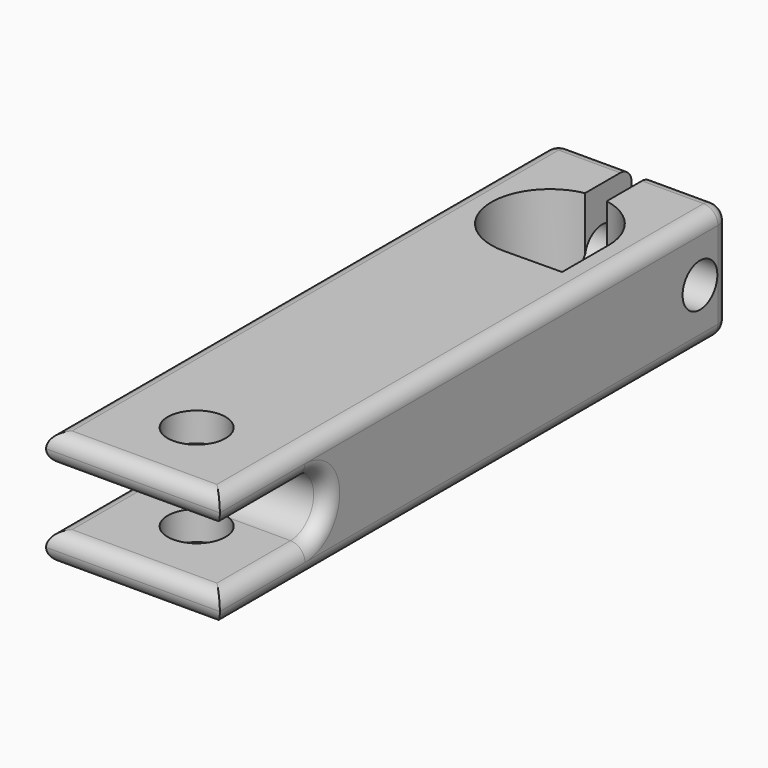
from build123d import *

# Parameters (mm, degrees)
F0_W      = 38.1
F0_H      = 139.7
F0_R      = 12.827
F1_DEPTH  = 25.4
F3_DEPTH  = 25.4
F4_R      = 4.7625
F5_DEPTH  = 127
F6_R      = 6.35
F7_DEPTH  = 50.8
F8_W      = 23.3431950331
F8_H      = 12.7
F9_DEPTH  = 76.2
F10_R     = 3.17499
F12_DEPTH = 25.4


# Not quite as in the source:
# - a fillet or chamfer is up to 0.001 mm smaller than in the source, because OpenCascade refuses the exact size


with BuildPart() as f1:
    # F0 (on Top) → F1 (new body)
    with BuildSketch(Plane.XY):
        with Locations((-13.4720488012, -10.8498208284)):
            Rectangle(F0_W, F0_H)
        with Locations((-13.4720488012, 33.6001791716)):
            Circle(F0_R, mode=Mode.SUBTRACT)
    extrude(amount=F1_DEPTH)

    # F2 (on face) → F3 (cut)
    with BuildSketch(Plane.XY.offset(25.4)):
        with BuildLine():
            Line((-11.0907988012, 46.2042093777), (-11.0907988012, 59.0001791716))
            Line((-11.0907988012, 59.0001791716), (-15.8532988012, 59.0001791716))
            Line((-15.8532988012, 59.0001791716), (-15.8532988012, 46.2042093777))
            ThreePointArc((-15.8532988012, 46.2042093777), (-13.4720488012, 46.4271791716), (-11.0907988012, 46.2042093777))
        make_face()
    extrude(amount=-F3_DEPTH, mode=Mode.SUBTRACT)

    # F4 (on face) → F5 (cut)
    with BuildSketch(Plane(origin=(-32.5220488012, 0, 0), x_dir=(0, -1, 0), z_dir=(-1, 0, 0))):
        with Locations((-50.9158676147, 12.7)):
            Circle(F4_R)
    extrude(amount=-F5_DEPTH, mode=Mode.SUBTRACT)

    # F6 (on face) → F7 (cut)
    with BuildSketch(Plane.XY.offset(25.4)):
        with Locations((-13.4720488012, -63.2373208284)):
            Circle(F6_R)
    extrude(amount=-F7_DEPTH, mode=Mode.SUBTRACT)

    # F8 (on face) → F9 (cut)
    with BuildSketch(Plane.YZ.offset(5.5779511988)):
        with Locations((-69.0282233119, 12.7)):
            Rectangle(F8_W, F8_H)
        with BuildLine():
            Line((-57.3566257954, 19.05), (-57.3566257954, 6.35))
            ThreePointArc((-57.3566257954, 6.35), (-51.0066257954, 12.7), (-57.3566257954, 19.05))
        make_face()
    extrude(amount=-F9_DEPTH, mode=Mode.SUBTRACT)

    # F10 (radius 3.175 in the source; OpenCascade refuses exactly that, so slightly less here)
    f10_edges = [f1.edges().sort_by_distance(p)[0] for p in [
        (5.577951, -69.028223, 19.05),
        (-13.472049, -80.699821, 6.35),
        (5.577951, -10.849821, 25.4),
        (-32.522049, -10.849821, 25.4),
        (-13.472049, -80.699821, 25.4),
        (5.577951, -10.849821, 0),
        (-13.472049, -80.699821, 0),
        (-24.187674, 59.000179, 25.4),
        (-2.756424, 59.000179, 25.4),
        (-32.522049, 59.000179, 12.7),
        (5.577951, 59.000179, 12.7),
        (-2.756424, 59.000179, 0),
        (-24.187674, 59.000179, 0),
        (-32.522049, -10.849821, 0),
        (-13.472049, -80.699821, 19.05),
        (-32.522049, -51.006626, 12.7),
        (-32.522049, -69.028223, 6.35),
        (-32.522049, -69.028223, 19.05),
    ]]
    fillet(f10_edges, radius=F10_R)

    # F11 (on face) → F12 (cut)
    with BuildSketch(Plane.XY.offset(25.4)):
        with BuildLine():
            Line((-0.6450488012, 20.9001791716), (-0.6450488012, 33.6001791716))
            ThreePointArc((-0.6450488012, 33.6001791716), (-4.3126364935, 24.6203631836), (-13.2180736983, 20.7756937765))
            Line((-13.2180736983, 20.7756937765), (-0.6450488012, 20.9001791716))
        make_face()
    extrude(amount=-F12_DEPTH, mode=Mode.SUBTRACT)


solid = f1.part
